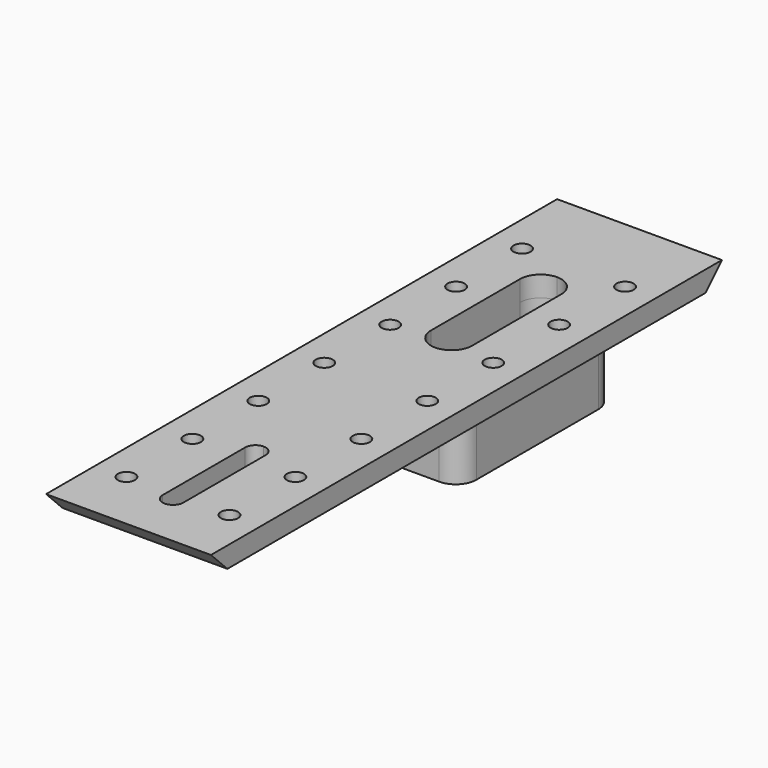
from build123d import *

# Parameters (mm, degrees)
F0_W      = 40
F0_H      = 155
F0_W_2    = 10
F0_H_2    = 37
F1_DEPTH  = 5
F2_R      = 4.99999
F3_W      = 20
F3_H      = 47
F4_DEPTH  = 20
F5_R      = 5
F6_SIZE   = 4.99999
F7_R      = 2.074
F8_DEPTH  = 25.001
F9_W      = 5
F9_H      = 30
F10_DEPTH = 25.001
F11_R     = 2.49999


# Not quite as in the source:
# - a fillet or chamfer is up to 0.001 mm smaller than in the source, because OpenCascade refuses the exact size
# - ends of sketch curves that miss each other by under 0.0002 mm in the source are joined


with BuildPart() as f1:
    # F0 (on Top) → F1 (new body)
    with BuildSketch(Plane.XY):
        with Locations((0, 20)):
            Rectangle(F0_W, F0_H)
        with Locations((0, 54)):
            Rectangle(F0_W_2, F0_H_2, mode=Mode.SUBTRACT)
    extrude(amount=F1_DEPTH)

    # F2 (radius 5 in the source; OpenCascade refuses exactly that, so slightly less here)
    f2_edges = [f1.edges().sort_by_distance(p)[0] for p in [
        (5, 72.5, 2.5),
        (-5, 72.5, 2.5),
        (5, 35.5, 2.5),
        (-5, 35.5, 2.5),
    ]]
    fillet(f2_edges, radius=F2_R)

    # F3 (on face) → F4 (join)
    with BuildSketch(Plane(origin=(0, 0, 0), x_dir=(1, 0, 0), z_dir=(0, 0, -1))):
        with Locations((0, -54)):
            Rectangle(F3_W, F3_H)
        with BuildLine():
            ThreePointArc((-1e-05, -72.5), (-3.5355368349, -71.0355368349), (-5, -67.50001))
            Line((-5, -67.50001), (-5, -40.49999))
            ThreePointArc((-5, -40.49999), (-3.5355368349, -36.9644631651), (-1e-05, -35.5))
            ThreePointArc((-1e-05, -35.5), (3.5355368349, -36.9644631651), (5, -40.49999))
            Line((5, -40.49999), (5, -67.50001))
            ThreePointArc((5, -67.50001), (3.5355368349, -71.0355368349), (-1e-05, -72.5))
        make_face(mode=Mode.SUBTRACT)
    extrude(amount=F4_DEPTH)

    # F5
    f5_edges = [f1.edges().sort_by_distance(p)[0] for p in [
        (-10, 30.5, -10),
        (10, 30.5, -10),
        (-10, 77.5, -10),
        (10, 77.5, -10),
    ]]
    fillet(f5_edges, radius=F5_R)

    # F6 (size 5 in the source; OpenCascade refuses exactly that, so slightly less here)
    f6_edges = [f1.edges().sort_by_distance(p)[0] for p in [
        (0, 97.5, 0),
        (0, -57.5, 0),
    ]]
    chamfer(f6_edges, length=F6_SIZE)

    # F7 (on face) → F8 (cut, through all)
    with BuildSketch(Plane.XY.offset(5)):
        with Locations((-12.5, -42.5)):
            Circle(F7_R)
        with Locations((12.5, -42.5)):
            Circle(F7_R)
        with Locations((-12.5, -22.5)):
            Circle(F7_R)
        with Locations((12.5, -22.5)):
            Circle(F7_R)
        with Locations((-12.5, -2.5)):
            Circle(F7_R)
        with Locations((12.5, -2.5)):
            Circle(F7_R)
        with Locations((-12.5, 17.5)):
            Circle(F7_R)
        with Locations((12.5, 17.5)):
            Circle(F7_R)
        with Locations((-12.5, 37.5)):
            Circle(F7_R)
        with Locations((12.5, 37.5)):
            Circle(F7_R)
        with Locations((12.5, 57.5)):
            Circle(F7_R)
        with Locations((-12.5, 57.5)):
            Circle(F7_R)
        with Locations((12.5, 77.5)):
            Circle(F7_R)
        with Locations((-12.5, 77.5)):
            Circle(F7_R)
    extrude(amount=-F8_DEPTH, mode=Mode.SUBTRACT)

    # F9 (on face) → F10 (cut, through all)
    with BuildSketch(Plane.XY.offset(5)):
        with Locations((0, -31.5)):
            Rectangle(F9_W, F9_H)
    extrude(amount=-F10_DEPTH, mode=Mode.SUBTRACT)

    # F11 (radius 2.5 in the source; OpenCascade refuses exactly that, so slightly less here)
    f11_edges = [f1.edges().sort_by_distance(p)[0] for p in [
        (-2.5, -46.5, 2.5),
        (2.5, -46.5, 2.5),
        (-2.5, -16.5, 2.5),
        (2.5, -16.5, 2.5),
    ]]
    fillet(f11_edges, radius=F11_R)


solid = f1.part
